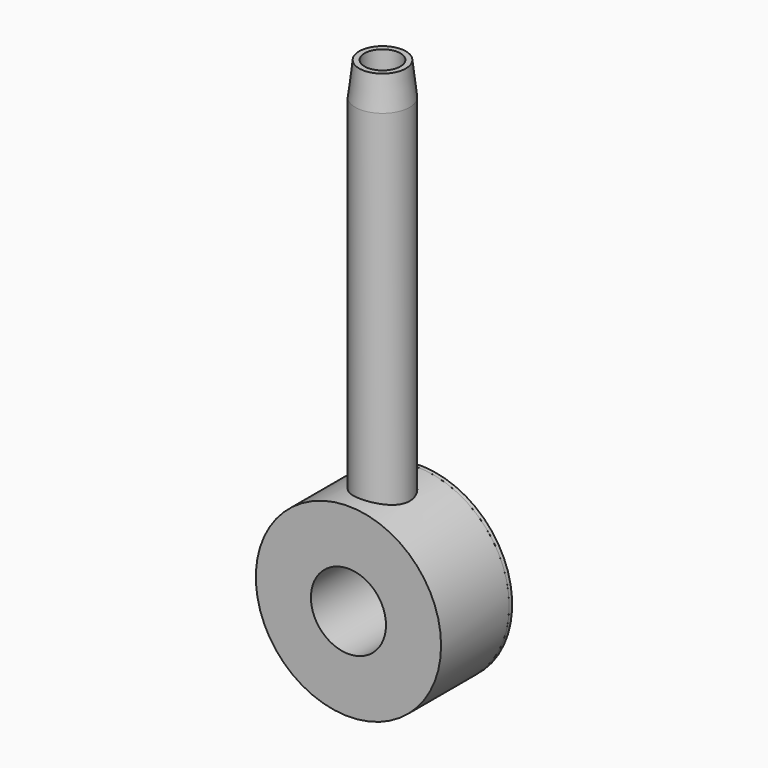
from build123d import *

# Parameters (mm, degrees)
F0_R          = 37
F0_R_2        = 15
F1_DEPTH      = 34
F2_R          = 23
F2_R_2        = 15
F3_DEPTH      = 1.5
F4_R          = 23
F4_R_2        = 20
F5_DEPTH      = 17
F8_END_RADIUS = 20
F7_R          = 7.15
F8_REACH      = 94.2242539419
F9_R          = 10.85
F10_DEPTH     = 10
F11_R         = 10.85
F11_R_2       = 7.15
F12_DEPTH     = 160
F13_SIZE2     = 13.16
F13_SIZE      = 1.5345
F14_R         = 37
F14_R_2       = 23
F15_DEPTH     = 1.5


with BuildPart() as f1:
    # F0 (on Front) → F1 (new body)
    with BuildSketch(Plane.XZ):
        Circle(F0_R)
        Circle(F0_R_2, mode=Mode.SUBTRACT)
    extrude(amount=F1_DEPTH)

    # F2 (on face) → F3 (cut)
    with BuildSketch(Plane(origin=(0, 0, 0), x_dir=(-1, 0, 0), z_dir=(0, 1, 0))):
        Circle(F2_R)
        Circle(F2_R_2, mode=Mode.SUBTRACT)
    extrude(amount=-F3_DEPTH, mode=Mode.SUBTRACT)

    # F4 (on face) → F5 (cut)
    with BuildSketch(Plane(origin=(0, 0, 0), x_dir=(-1, 0, 0), z_dir=(0, 1, 0))):
        Circle(F4_R)
        Circle(F4_R_2, mode=Mode.SUBTRACT)
    extrude(amount=-F5_DEPTH, mode=Mode.SUBTRACT)

    f8_end = (Plane.ZX.offset(-9.25) * Cylinder(F8_END_RADIUS, 408.5212231395, mode=Mode.PRIVATE)).faces().sort_by_distance((20, -9.25, 0))[0]
    # F7 (on offset) → F8 (cut, up to the whole of a round face its end follows)
    with BuildSketch(Plane.XY.offset(37)):
        with Locations((0, -17)):
            Circle(F7_R)
    f8_long = extrude(amount=-F8_REACH, mode=Mode.PRIVATE)
    add(split(f8_long, bisect_by=f8_end, keep=Keep.ALL, mode=Mode.PRIVATE).solids().sort_by_distance((0, -17, 37))[0], mode=Mode.SUBTRACT)

    # F9 (on offset) → F10 (cut)
    with BuildSketch(Plane.XY.offset(37)):
        with Locations((0, -17)):
            Circle(F9_R)
    extrude(amount=-F10_DEPTH, mode=Mode.SUBTRACT)


with BuildPart() as f12:
    # F11 (on face) → F12 (new body)
    with BuildSketch(Plane.XY.offset(27)):
        with Locations((0, -17)):
            Circle(F11_R)
        with Locations((0, -17)):
            Circle(F11_R_2, mode=Mode.SUBTRACT)
    extrude(amount=F12_DEPTH)

    # F13
    f13_edges = [f12.edges().sort_by_distance(p)[0] for p in [
        (-10.85, -17, 187),
    ]]
    f13_side = f12.faces().sort_by_distance((-10.543116, -17, 187))[0]
    chamfer(f13_edges, length=F13_SIZE, length2=F13_SIZE2, reference=f13_side)


with BuildPart() as f15:
    # F14 (on face) → F15 (new body)
    with BuildSketch(Plane(origin=(0, 0, 0), x_dir=(-1, 0, 0), z_dir=(0, 1, 0))):
        Circle(F14_R)
        Circle(F14_R_2, mode=Mode.SUBTRACT)
    extrude(amount=F15_DEPTH)


solid = Compound([f1.part, f12.part, f15.part])
